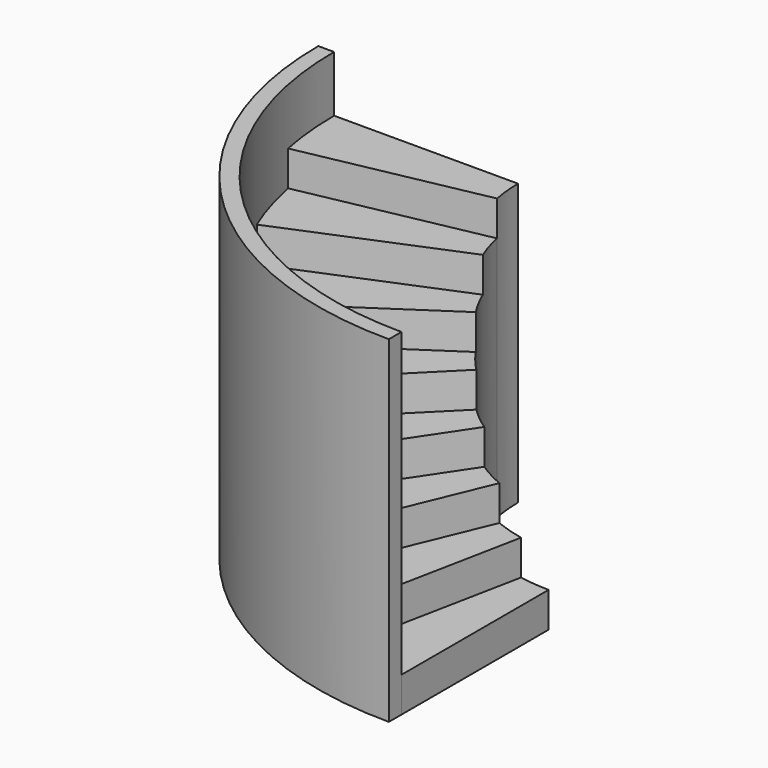
from build123d import *

# Parameters (mm, degrees)
F10_DEPTH = 254
F11_DEPTH = 508
F12_DEPTH = 762
F13_DEPTH = 1016
F14_DEPTH = 1270
F15_DEPTH = 1524
F16_DEPTH = 1778
F17_DEPTH = 2032
F19_DEPTH = 2438.4


# Not quite as in the source:
# - a variable given as a bare number and used for a length is read in inches; the dataset says mm whatever the document's units were


with BuildPart() as f10:
    # F2 (on Top) → F10 (new body)
    with BuildSketch(Plane.XY):
        with BuildLine():
            Line((-979.52713178, -1331.3833333333), (-979.52713178, 0))
            ThreePointArc((-979.52713178, 0), (-1088.0337397438, 5.3305878284), (-1195.4953697572, 21.271014839))
            Line((-1195.4953697572, 21.271014839), (-1455.2353729841, -1284.5301610686))
            ThreePointArc((-1455.2353729841, -1284.5301610686), (-1218.5321267596, -1319.6417708508), (-979.52713178, -1331.3833333333))
        make_face()
    extrude(amount=F10_DEPTH)

    # F3 (on Top) → F11 (join)
    with BuildSketch(Plane.XY):
        with BuildLine():
            Line((-1455.2353729841, -1284.5301610686), (-1195.4953697572, 21.271014839))
            ThreePointArc((-1195.4953697572, 21.271014839), (-1300.8771075786, 47.6677660055), (-1403.1640694653, 84.2666261845))
            Line((-1403.1640694653, 84.2666261845), (-1912.662413259, -1145.7711854089))
            ThreePointArc((-1912.662413259, -1145.7711854089), (-1687.3572887973, -1226.3866479828), (-1455.2353729841, -1284.5301610686))
        make_face()
    extrude(amount=F11_DEPTH)

    # F4 (on Top) → F12 (join)
    with BuildSketch(Plane.XY):
        with BuildLine():
            Line((-1912.662413259, -1145.7711854089), (-1403.1640694653, 84.2666261845))
            ThreePointArc((-1403.1640694653, 84.2666261845), (-1501.3711760586, 130.7151283453), (-1594.5526392366, 186.5659480209))
            Line((-1594.5526392366, 186.5659480209), (-2334.229587975, -920.4388359719))
            ThreePointArc((-2334.229587975, -920.4388359719), (-2128.9809348565, -1043.4601443204), (-1912.662413259, -1145.7711854089))
        make_face()
    extrude(amount=F12_DEPTH)

    # F5 (on Top) → F13 (join)
    with BuildSketch(Plane.XY):
        with BuildLine():
            Line((-2334.229587975, -920.4388359719), (-1594.5526392366, 186.5659480209))
            ThreePointArc((-1594.5526392366, 186.5659480209), (-1681.8110705705, 251.2812112866), (-1762.3061236665, 324.2376747801))
            Line((-1762.3061236665, 324.2376747801), (-2703.7363070253, -617.1925085786))
            ThreePointArc((-2703.7363070253, -617.1925085786), (-2526.4317158846, -777.892022813), (-2334.229587975, -920.4388359719))
        make_face()
    extrude(amount=F13_DEPTH)

    # F6 (on Top) → F14 (join)
    with BuildSketch(Plane.XY):
        with BuildLine():
            Line((-2703.7363070253, -617.1925085786), (-1762.3061236665, 324.2376747801))
            ThreePointArc((-1762.3061236665, 324.2376747801), (-1835.2625871601, 404.7327278761), (-1899.9778504258, 491.9911592101))
            Line((-1899.9778504258, 491.9911592101), (-3006.9826344185, -247.6857895283))
            ThreePointArc((-3006.9826344185, -247.6857895283), (-2864.4358212597, -439.887917438), (-2703.7363070253, -617.1925085786))
        make_face()
    extrude(amount=F14_DEPTH)

    # F7 (on Top) → F15 (join)
    with BuildSketch(Plane.XY):
        with BuildLine():
            Line((-3006.9826344185, -247.6857895283), (-1899.9778504258, 491.9911592101))
            ThreePointArc((-1899.9778504258, 491.9911592101), (-1955.8286701014, 585.172622388), (-2002.2771722622, 683.3797289813))
            Line((-2002.2771722622, 683.3797289813), (-3232.3149838555, 173.8813851876))
            ThreePointArc((-3232.3149838555, 173.8813851876), (-3130.003942767, -42.4371364098), (-3006.9826344185, -247.6857895283))
        make_face()
    extrude(amount=F15_DEPTH)

    # F8 (on Top) → F16 (join)
    with BuildSketch(Plane.XY):
        with BuildLine():
            Line((-3232.3149838555, 173.8813851876), (-2002.2771722622, 683.3797289813))
            ThreePointArc((-2002.2771722622, 683.3797289813), (-2038.8760324411, 785.666690868), (-2065.2727836077, 891.0484286894))
            Line((-2065.2727836077, 891.0484286894), (-3371.0739595152, 631.3084254625))
            ThreePointArc((-3371.0739595152, 631.3084254625), (-3312.9304464294, 399.1865096494), (-3232.3149838555, 173.8813851876))
        make_face()
    extrude(amount=F16_DEPTH)

    # F9 (on Top) → F17 (join)
    with BuildSketch(Plane.XY):
        with BuildLine():
            Line((-3371.0739595152, 631.3084254625), (-2065.2727836077, 891.0484286894))
            ThreePointArc((-2065.2727836077, 891.0484286894), (-2081.2132106182, 998.5100587028), (-2086.5437984467, 1107.0166666667))
            Line((-2086.5437984467, 1107.0166666667), (-3417.92713178, 1107.0166666667))
            ThreePointArc((-3417.92713178, 1107.0166666667), (-3406.1855692975, 868.0116716871), (-3371.0739595152, 631.3084254625))
        make_face()
    extrude(amount=F17_DEPTH)


with BuildPart() as f19:
    # F18 (on Top) → F19 (new body)
    with BuildSketch(Plane.XY):
        with BuildLine():
            ThreePointArc((-979.52713178, -1331.3833333333), (-2703.7363070253, -617.1925085786), (-3417.92713178, 1107.0166666667))
            Line((-3417.92713178, 1107.0166666667), (-3532.22713178, 1107.0166666667))
            ThreePointArc((-3532.22713178, 1107.0166666667), (-2784.5586121149, -698.0148136682), (-979.52713178, -1445.6833333333))
            Line((-979.52713178, -1445.6833333333), (-979.52713178, -1331.3833333333))
        make_face()
    extrude(amount=F19_DEPTH)


solid = Compound([f10.part, f19.part])
